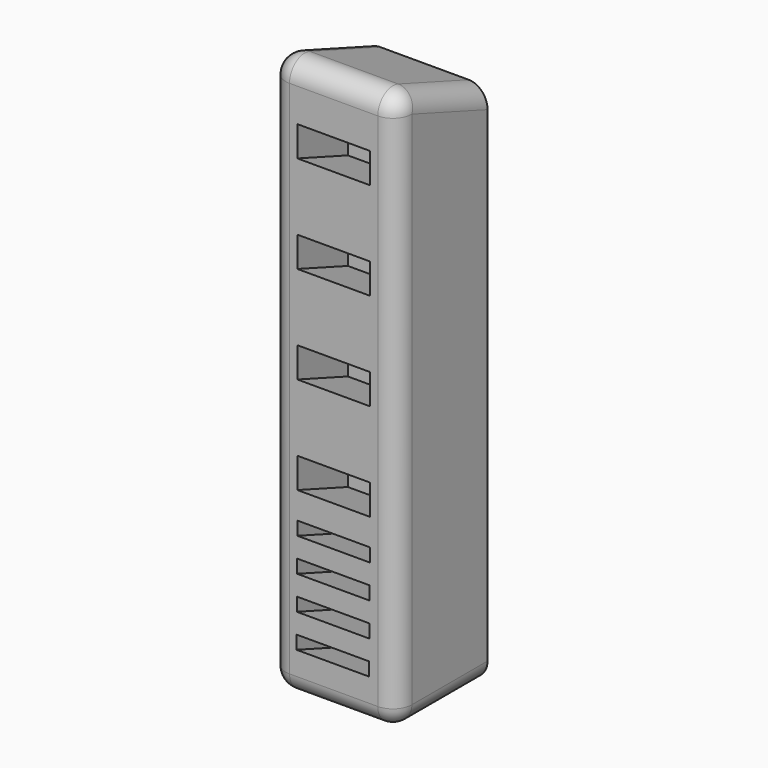
from build123d import *
from build123d import SkipClean  # not in build123d's __all__

# Parameters (mm, degrees)
F0_W      = 20
F0_H      = 90
F1_DEPTH  = 18
F4_W      = 11.5
F4_H      = 4.5
F4_H_2    = 2
F6_REACH  = 51.4753785472
F8_W      = 43.5633249581
F8_H      = 43.13050583
F9_DEPTH  = 16.4
F10_R     = 3
F12_DEPTH = 7
F13_DEPTH = 1


with BuildPart() as f1:
    # F0 (on Front) → F1 (new body)
    with BuildSketch(Plane.XZ):
        Rectangle(F0_W, F0_H)
    extrude(amount=F1_DEPTH)

    f6_end = Plane(origin=(0, -8, 0), x_dir=(0, 0, -1), z_dir=(0, -1, 0))
    # F4 (on face) → F6 (cut, up to a plane its end follows)
    with BuildSketch(Plane(origin=(0, -30.357121206, 11.049088517), x_dir=(-1, 0, 0), z_dir=(0, 0.9396926208, -0.3420201433))):
        with Locations((0, 24.6185707509)):
            Rectangle(F4_W, F4_H)
        with Locations((0, 10.1185707509)):
            Rectangle(F4_W, F4_H)
        with Locations((0, -4.3814292491)):
            Rectangle(F4_W, F4_H)
        with Locations((0, -18.8814292491)):
            Rectangle(F4_W, F4_H)
        with Locations((0, -26.1314292491)):
            Rectangle(F4_W, F4_H_2)
        with Locations((0.0476672364, -31.1312020274)):
            Rectangle(F4_W, F4_H_2)
        with Locations((0.0953344728, -36.1309748057)):
            Rectangle(F4_W, F4_H_2)
        with Locations((0.1430017093, -41.130747584)):
            Rectangle(F4_W, F4_H_2)
    f6_long = extrude(amount=F6_REACH, mode=Mode.PRIVATE)
    add(split(f6_long, bisect_by=f6_end, keep=Keep.TOP, mode=Mode.PRIVATE), mode=Mode.SUBTRACT)

    # F8 (on offset) → F9 (cut)
    with BuildSketch(Plane(origin=(0, 12.2677737091, 33.7054312527), x_dir=(1, 0, 0), z_dir=(0, -0.3420201433, -0.9396926208))):
        with Locations((0, 21.565252915)):
            Rectangle(F8_W, F8_H)
    extrude(amount=-F9_DEPTH, mode=Mode.SUBTRACT)

    # F10
    f10_edges = [f1.edges().sort_by_distance(p)[0] for p in [
        (-10, -18, -0.139),
        (0, -18, 44.722),
        (10, -18, -0.139),
        (0, -18, -45),
        (-10, -9, 41.446268),
        (10, -9, 41.446268),
        (-10, -9, -45),
        (10, -9, -45),
    ]]
    fillet(f10_edges, radius=F10_R)

    # F11 (on face) → F12 (cut)
    with BuildSketch(Plane(origin=(0, 0, 0), x_dir=(-1, 0, 0), z_dir=(0, 1, 0))):
        with BuildLine():
            ThreePointArc((-5.25, 20), (0, 14.75), (5.25, 20))
            ThreePointArc((5.25, 20), (4.9157552788, 21.8433258091), (3.9555809377, 23.4519385054))
            ThreePointArc((3.9555809377, 23.4519385054), (0, 25.25), (-3.9555809377, 23.4519385054))
            ThreePointArc((-3.9555809377, 23.4519385054), (-4.9157552788, 21.8433258091), (-5.25, 20))
        make_face()
        with BuildLine():
            ThreePointArc((3.9555809377, 23.4519385054), (4.9157552788, 21.8433258091), (5.25, 20))
            Line((5.25, 20), (5.25, 32.8980128765))
            ThreePointArc((5.25, 32.8980128765), (4.6642135624, 34.3122264389), (3.25, 34.8980128765))
            Line((3.25, 34.8980128765), (-3.25, 34.8980128765))
            ThreePointArc((-3.25, 34.8980128765), (-4.6642135624, 34.3122264389), (-5.25, 32.8980128765))
            Line((-5.25, 32.8980128765), (-5.25, 20))
            ThreePointArc((-5.25, 20), (-4.9157552788, 21.8433258091), (-3.9555809377, 23.4519385054))
            Line((-3.9555809377, 23.4519385054), (-3.9555809377, 31.6754657328))
            ThreePointArc((-3.9555809377, 31.6754657328), (-3.3697945001, 33.0896792952), (-1.9555809377, 33.6754657328))
            Line((-1.9555809377, 33.6754657328), (1.9555809377, 33.6754657328))
            ThreePointArc((1.9555809377, 33.6754657328), (3.3697945001, 33.0896792952), (3.9555809377, 31.6754657328))
            Line((3.9555809377, 31.6754657328), (3.9555809377, 23.4519385054))
        make_face()
        with BuildLine():
            ThreePointArc((-3.9555809377, 23.4519385054), (0, 25.25), (3.9555809377, 23.4519385054))
            Line((3.9555809377, 23.4519385054), (3.9555809377, 31.6754657328))
            ThreePointArc((3.9555809377, 31.6754657328), (3.3697945001, 33.0896792952), (1.9555809377, 33.6754657328))
            Line((1.9555809377, 33.6754657328), (-1.9555809377, 33.6754657328))
            ThreePointArc((-1.9555809377, 33.6754657328), (-3.3697945001, 33.0896792952), (-3.9555809377, 31.6754657328))
            Line((-3.9555809377, 31.6754657328), (-3.9555809377, 23.4519385054))
        make_face()
    extrude(amount=-F12_DEPTH, mode=Mode.SUBTRACT)

    # F11 (on face) → F13 (join)
    with BuildSketch(Plane(origin=(0, 0, 0), x_dir=(-1, 0, 0), z_dir=(0, 1, 0))):
        with BuildLine():
            ThreePointArc((3.9555809377, 23.4519385054), (4.9157552788, 21.8433258091), (5.25, 20))
            Line((5.25, 20), (5.25, 32.8980128765))
            ThreePointArc((5.25, 32.8980128765), (4.6642135624, 34.3122264389), (3.25, 34.8980128765))
            Line((3.25, 34.8980128765), (-3.25, 34.8980128765))
            ThreePointArc((-3.25, 34.8980128765), (-4.6642135624, 34.3122264389), (-5.25, 32.8980128765))
            Line((-5.25, 32.8980128765), (-5.25, 20))
            ThreePointArc((-5.25, 20), (-4.9157552788, 21.8433258091), (-3.9555809377, 23.4519385054))
            Line((-3.9555809377, 23.4519385054), (-3.9555809377, 31.6754657328))
            ThreePointArc((-3.9555809377, 31.6754657328), (-3.3697945001, 33.0896792952), (-1.9555809377, 33.6754657328))
            Line((-1.9555809377, 33.6754657328), (1.9555809377, 33.6754657328))
            ThreePointArc((1.9555809377, 33.6754657328), (3.3697945001, 33.0896792952), (3.9555809377, 31.6754657328))
            Line((3.9555809377, 31.6754657328), (3.9555809377, 23.4519385054))
        make_face()
    with SkipClean():  # cleaning this boolean's faces spoils the solid; the shape is the same uncleaned
        extrude(amount=-F13_DEPTH)


solid = f1.part
